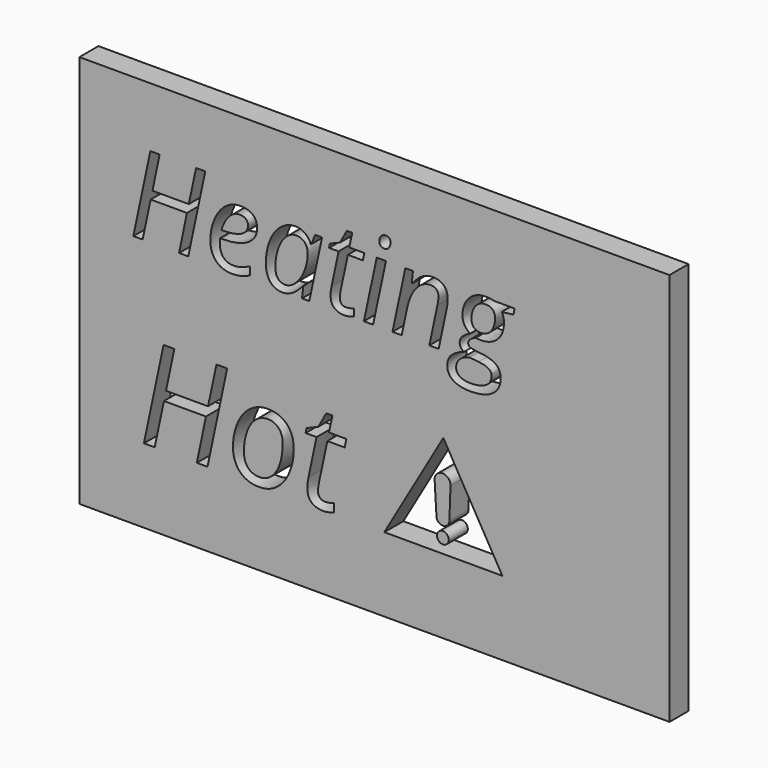
from build123d import *

# Parameters (mm, degrees)
F0_W           = 76.2
F0_H           = 3.0734
F1_DEPTH       = 50.8
F2_TEXT_SIZE   = 14.5402504472
F2_R           = 0.762
F2_TEXT_SIZE_2 = 16.8202426865
F3_DEPTH       = 25.4


# Not quite as in the source:
# - Text() gives the source's letters only with a copy of the font that has no kerning and outlines rounded to 1/6400 em; it was checked with that copy


with BuildPart() as f1:
    # F0 (on Top) → F1 (new body)
    with BuildSketch(Plane.XY):
        Rectangle(F0_W, F0_H)
    extrude(amount=F1_DEPTH)

    # F2 (on face) → F3 (cut)
    with BuildSketch(Plane.XZ.offset(1.5367)):
        with Locations((-31.75, 32.711019678)):
            Text('Heating', F2_TEXT_SIZE, font='Open Sans', font_style=FontStyle.ITALIC, text_align=(TextAlign.LEFT, TextAlign.BOTTOM))
        Polygon((8.89, 22.7899297779), (1.27, 9.5917026242), (16.51, 9.5917026242), align=None)
        with Locations((8.8331749315, 11.419244998)):
            Circle(F2_R, mode=Mode.SUBTRACT)
        with BuildLine():
            Line((7.9965411264, 13.7103661618), (7.7578957783, 17.7673532703))
            ThreePointArc((7.7578957783, 17.7673532703), (8.8418110619, 18.7255223116), (9.8184813528, 17.6582475593))
            Line((9.8184813528, 17.6582475593), (9.673431564, 13.5968368982))
            ThreePointArc((9.673431564, 13.5968368982), (8.7763814051, 12.7879739328), (7.9965411264, 13.7103661618))
        make_face(mode=Mode.SUBTRACT)
        with Locations((-30.48, 9.6012)):
            Text('Hot', F2_TEXT_SIZE_2, font='Open Sans', font_style=FontStyle.ITALIC, text_align=(TextAlign.LEFT, TextAlign.BOTTOM))
    extrude(amount=-F3_DEPTH, mode=Mode.SUBTRACT)


solid = f1.part
